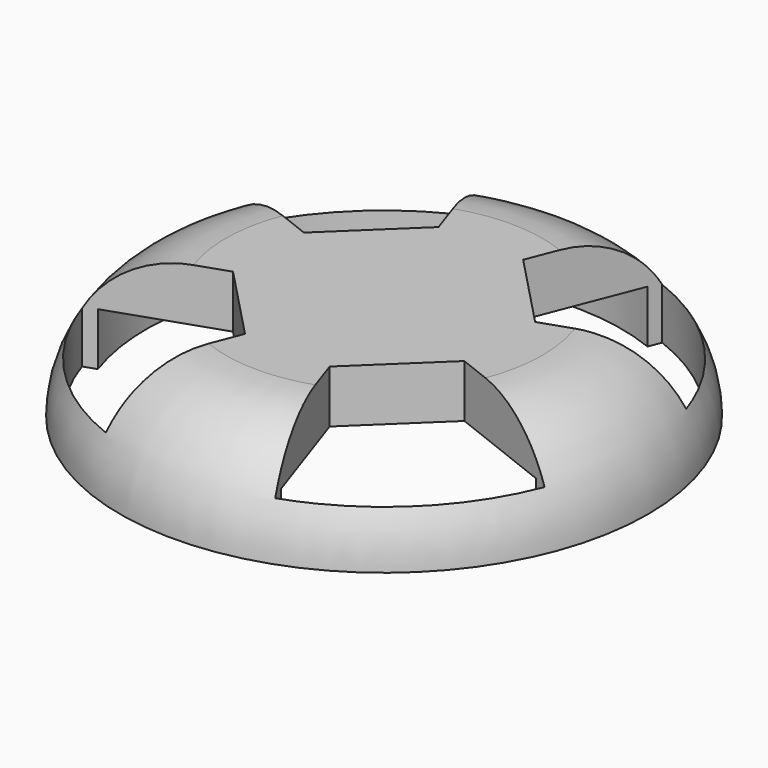
from build123d import *

# Parameters (mm, degrees)
F0_R     = 50
F1_DEPTH = 20
F2_R     = 19.99999
F3_R     = 45
F4_DEPTH = 10
F6_DEPTH = 25


# Not quite as in the source:
# - a fillet or chamfer is up to 0.001 mm smaller than in the source, because OpenCascade refuses the exact size


with BuildPart() as f1:
    # F0 (on Top) → F1 (new body)
    with BuildSketch(Plane.XY):
        Circle(F0_R)
    extrude(amount=F1_DEPTH)

    # F2 (radius 20 in the source; OpenCascade refuses exactly that, so slightly less here)
    f2_edges = [f1.edges().sort_by_distance(p)[0] for p in [
        (-50, 0, 20),
    ]]
    fillet(f2_edges, radius=F2_R)

    # F3 (on face) → F4 (cut)
    with BuildSketch(Plane(origin=(0, 0, 0), x_dir=(1, 0, 0), z_dir=(0, 0, -1))):
        Circle(F3_R)
    extrude(amount=-F4_DEPTH, mode=Mode.SUBTRACT)

    # F5 (on face) → F6 (cut)
    with BuildSketch(Plane.XY.offset(20)):
        with BuildLine():
            Line((-22.4775391325, -7.6695980696), (-44.9550782649, -15.3391961392))
            ThreePointArc((-44.9550782649, -15.3391961392), (-34.3172747897, -32.8416602961), (-17.2989432787, -44.2379538568))
            Line((-17.2989432787, -44.2379538568), (-8.6494716394, -22.1189769284))
            Line((-8.6494716394, -22.1189769284), (-22.4775391325, -7.6695980696))
        make_face()
        with BuildLine():
            Line((-7.6695980696, 22.4775391325), (-15.3391961392, 44.9550782649))
            ThreePointArc((-15.3391961392, 44.9550782649), (-32.8416602961, 34.3172747897), (-44.2379538568, 17.2989432787))
            Line((-44.2379538568, 17.2989432787), (-22.1189769284, 8.6494716394))
            Line((-22.1189769284, 8.6494716394), (-7.6695980696, 22.4775391325))
        make_face()
        with BuildLine():
            Line((22.4775391325, 7.6695980696), (44.9550782649, 15.3391961392))
            ThreePointArc((44.9550782649, 15.3391961392), (34.3172747897, 32.8416602961), (17.2989432787, 44.2379538568))
            Line((17.2989432787, 44.2379538568), (8.6494716394, 22.1189769284))
            Line((8.6494716394, 22.1189769284), (22.4775391325, 7.6695980696))
        make_face()
        with BuildLine():
            Line((7.6695980696, -22.4775391325), (15.3391961392, -44.9550782649))
            ThreePointArc((15.3391961392, -44.9550782649), (32.8416602961, -34.3172747897), (44.2379538568, -17.2989432787))
            Line((44.2379538568, -17.2989432787), (22.1189769284, -8.6494716394))
            Line((22.1189769284, -8.6494716394), (7.6695980696, -22.4775391325))
        make_face()
    extrude(amount=-F6_DEPTH, mode=Mode.SUBTRACT)


solid = f1.part
